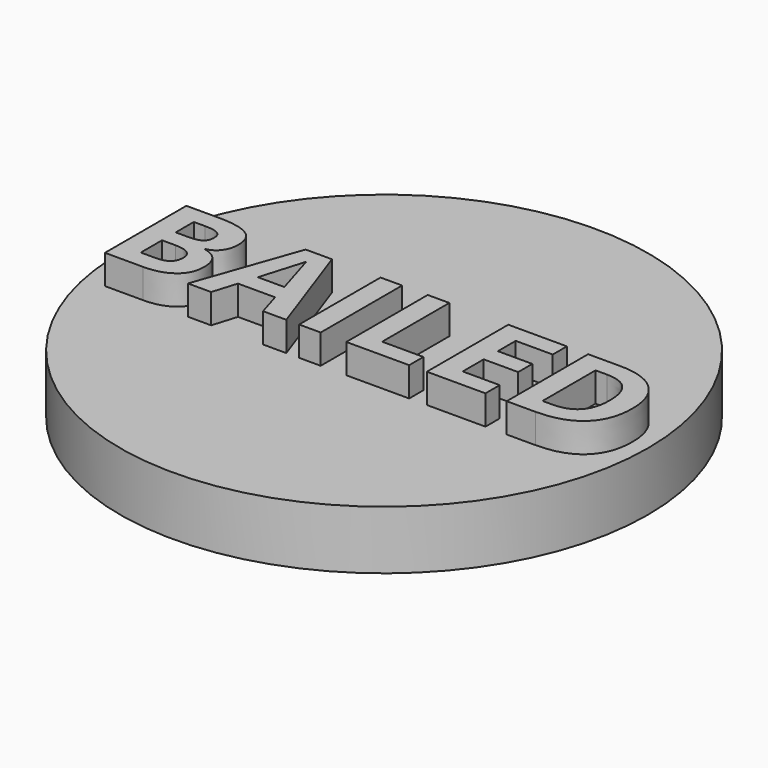
from build123d import *

# Parameters (mm, degrees)
F0_R         = 9
F1_DEPTH     = 2
F2_TEXT_SIZE = 4.8611111111
F3_DEPTH     = 1


# Not quite as in the source:
# - Text() gives the source's letters only with a copy of the font that has no kerning and outlines rounded to 1/6400 em; it was checked with that copy


with BuildPart() as f1:
    # F0 (on Top) → F1 (new body)
    with BuildSketch(Plane.XY):
        with Locations((-38.8579405844, 55.6978173554)):
            Circle(F0_R)
    extrude(amount=F1_DEPTH)

    # F2 (on face) → F3 (join)
    with BuildSketch(Plane.XY.offset(2)):
        with Locations((-47.4231505456, 53.9612043488)):
            Text('BAILED', F2_TEXT_SIZE, font='Open Sans', font_style=FontStyle.BOLD, text_align=(TextAlign.LEFT, TextAlign.BOTTOM))
    extrude(amount=F3_DEPTH)


solid = f1.part
